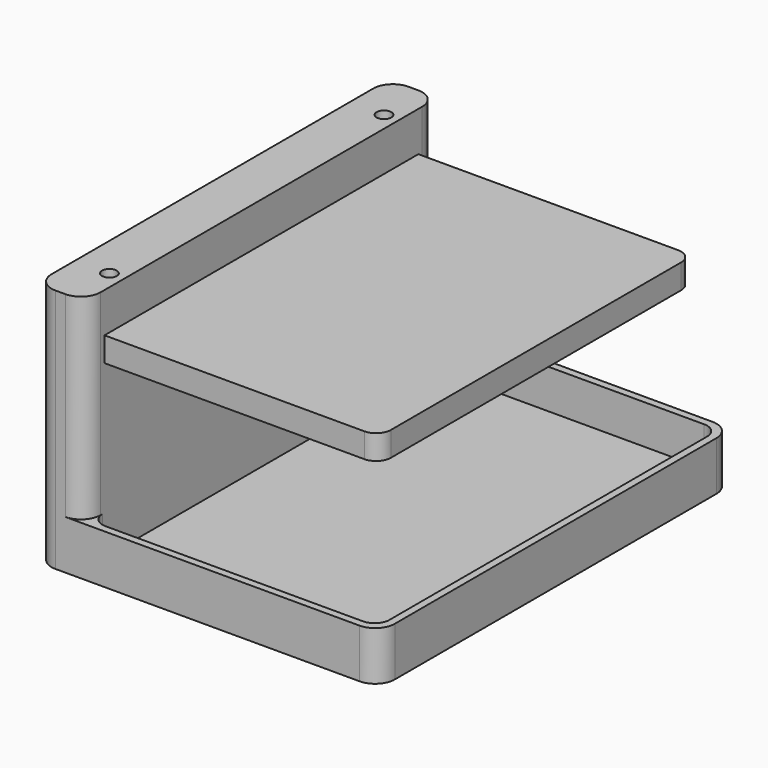
from build123d import *

# Parameters (mm, degrees)
F1_DEPTH      = 45
F1_DEPTH_BACK = 45
F2_W          = 67
F2_H          = 5
F3_DEPTH      = 40
F3_DEPTH_BACK = 40
F5_R          = 1.5
F6_DEPTH      = 30
F8_DEPTH      = 8
F9_R          = 4
F10_T1_DEPTH  = 20
F10_T3_DEPTH  = 16.1803398875


# Not quite as in the source:
# - a fillet or chamfer that OpenCascade refuses, or shapes differently, is made with other operations: its cross-section is extruded or revolved along the edge and cut away or added


with BuildPart() as f1:
    # F0 (on Front) → F1 (new body, two sides)
    with BuildSketch(Plane.XZ) as f1_sk:
        Polygon((0, 50), (0, 0), (70, 0), (70, 10), (10, 10), (10, 50), align=None)
    extrude(amount=F1_DEPTH)
    extrude(f1_sk.sketch, amount=-F1_DEPTH_BACK)

    # F2 (on Front) → F3 (join, two sides)
    with BuildSketch(Plane.XZ) as f3_sk:
        with Locations((32.5, 39.3734816462)):
            Rectangle(F2_W, F2_H)
    extrude(amount=-F3_DEPTH)
    extrude(f3_sk.sketch, amount=F3_DEPTH_BACK)

    # F5 (on offset) → F6 (cut)
    with BuildSketch(Plane.XY.offset(55)):
        with Locations((7, -35)):
            Circle(F5_R)
        with Locations((7, 35)):
            Circle(F5_R)
    extrude(amount=-F6_DEPTH, mode=Mode.SUBTRACT)

    # F7 (on face) → F8 (cut)
    with BuildSketch(Plane.XY.offset(10)):
        with BuildLine():
            ThreePointArc((68.5, 40.5), (67.6213203436, 42.6213203436), (65.5, 43.5))
            Line((65.5, 43.5), (13, 43.5))
            ThreePointArc((13, 43.5), (10.8786796564, 42.6213203436), (10, 40.5))
            Line((10, 40.5), (10, -40.5))
            ThreePointArc((10, -40.5), (10.8786796564, -42.6213203436), (13, -43.5))
            Line((13, -43.5), (65.5, -43.5))
            ThreePointArc((65.5, -43.5), (67.6213203436, -42.6213203436), (68.5, -40.5))
            Line((68.5, -40.5), (68.5, 40.5))
        make_face()
    extrude(amount=-F8_DEPTH, mode=Mode.SUBTRACT)

    # F9
    f9_edges = [f1.edges().sort_by_distance(p)[0] for p in [
        (70, -45, 5),
        (70, 45, 5),
        (0, -45, 25),
        (0, 45, 25),
        (10, -45, 30),
        (10, 45, 30),
    ]]
    fillet(f9_edges, radius=F9_R)

    # F10: fillet of radius 3 on 4 edges, made by hand

    # F10_s2 → F10_t1 (cut)
    with BuildSketch(Plane.XY.offset(29.3734816462)):
        with BuildLine():
            ThreePointArc((63, -40), (65.1213203436, -39.1213203436), (66, -37))
            Line((66, -37), (66, -40))
            Line((66, -40), (63, -40))
        make_face()
        with BuildLine():
            ThreePointArc((63, 40), (65.1213203436, 39.1213203436), (66, 37))
            Line((66, 37), (66, 40))
            Line((66, 40), (63, 40))
        make_face()
    extrude(amount=F10_T1_DEPTH, mode=Mode.SUBTRACT)

    # F10_s4 → F10_t3 (cut)
    with BuildSketch(Plane.XY.offset(31.2833117024)):
        with BuildLine():
            ThreePointArc((0, 40), (-0.7386127875, 38.9886768939), (-1, 37.7639320225))
            Line((-1, 37.7639320225), (-1, 40))
            Line((-1, 40), (0, 40))
        make_face()
        with BuildLine():
            ThreePointArc((0, -40), (-0.7386127875, -38.9886768939), (-1, -37.7639320225))
            Line((-1, -37.7639320225), (-1, -40))
            Line((-1, -40), (0, -40))
        make_face()
    extrude(amount=F10_T3_DEPTH, mode=Mode.SUBTRACT)


solid = f1.part
